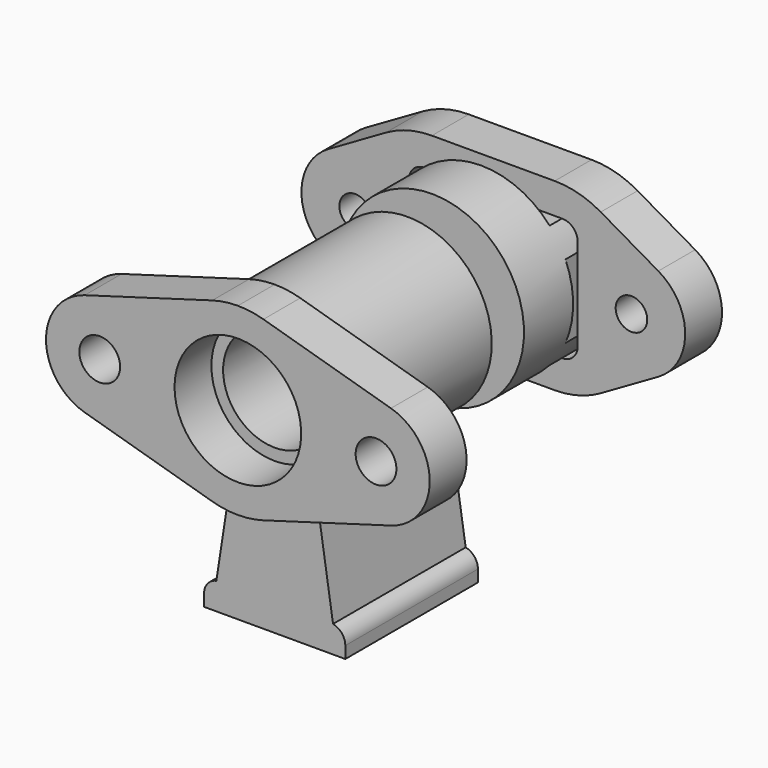
from build123d import *

# Parameters (mm, degrees)
F0_R      = 10.668
F1_DEPTH  = 34.29
F2_R      = 9.4615
F3_DEPTH  = 4.064
F5_D      = 6.5278
F5_DEPTH  = 19.05
F5_TIP    = 1.9611489744
F7_DEPTH  = 9.525
F8_D      = 26.19502
F9_D      = 8.4328
F11_R     = 19.05
F11_R_2   = 10.7823
F12_DEPTH = 25.4
F14_DEPTH = 12.7
F16_DEPTH = 9.525
F17_D     = 6.5278


# Not quite as in the source:
# - a pattern or mirror of a feature is missing from the dataset's text; its kind, count and spacing are read off the source's solid


with BuildPart() as f1:
    # F0 (on Front) → F1 (new body)
    with BuildSketch(Plane.XZ):
        with BuildLine():
            Line((12.065, -38.8341331818), (8.4555263158, -15.2788409565))
            ThreePointArc((8.4555263158, -15.2788409565), (0, 17.4625), (-8.4555263158, -15.2788409565))
            Line((-8.4555263158, -15.2788409565), (-12.065, -38.8341331818))
            ThreePointArc((-12.065, -38.8341331818), (-13.8893444248, -39.9369388409), (-14.605, -41.9449851551))
            Line((-14.605, -41.9449851551), (-14.605, -44.3992))
            Line((-14.605, -44.3992), (14.605, -44.3992))
            Line((14.605, -44.3992), (14.605, -41.9449851551))
            ThreePointArc((14.605, -41.9449851551), (13.8893444248, -39.9369388409), (12.065, -38.8341331818))
        make_face()
        Circle(F0_R, mode=Mode.SUBTRACT)
    extrude(amount=F1_DEPTH)

    # F2 (on face) → F3 (join)
    with BuildSketch(Plane(origin=(0, 0, -44.3992), x_dir=(1, 0, 0), z_dir=(0, 0, -1))):
        with Locations((0, 17.145)):
            Circle(F2_R)
    extrude(amount=F3_DEPTH)

    # F5
    with Locations(Plane(origin=(0, 0, -48.4632), x_dir=(1, 0, 0), z_dir=(0, 0, -1))):
        with Locations((0, 17.145)):
            Hole(F5_D / 2, depth=F5_DEPTH)
            with Locations((0, 0, -(F5_DEPTH + F5_TIP / 2))):  # 118° drill point
                Cone(0, F5_D / 2, F5_TIP, mode=Mode.SUBTRACT)


with BuildPart() as f7:
    # F6 (on face) → F7 (new body)
    with BuildSketch(Plane.XZ.offset(34.29)):
        with BuildLine():
            Line((5.2916666667, -18.300294093), (31.6618055556, -10.6751715542))
            ThreePointArc((31.6618055556, -10.6751715542), (39.6875, 0), (31.6618055556, 10.6751715542))
            Line((31.6618055556, 10.6751715542), (5.2916666667, 18.300294093))
            ThreePointArc((5.2916666667, 18.300294093), (2.6722553704, 18.861642326), (0, 19.05))
            ThreePointArc((0, 19.05), (-2.6722553704, 18.861642326), (-5.2916666667, 18.300294093))
            Line((-5.2916666667, 18.300294093), (-31.6618055556, 10.6751715542))
            ThreePointArc((-31.6618055556, 10.6751715542), (-39.6875, 0), (-31.6618055556, -10.6751715542))
            Line((-31.6618055556, -10.6751715542), (-5.2916666667, -18.300294093))
            ThreePointArc((-5.2916666667, -18.300294093), (-2.6722553704, -18.861642326), (0, -19.05))
            ThreePointArc((0, -19.05), (2.6722553704, -18.861642326), (5.2916666667, -18.300294093))
        make_face()
    extrude(amount=F7_DEPTH)

    # F8 (through all)
    with Locations(Plane(origin=(0, -34.29, 0), x_dir=(1, 0, 0), z_dir=(0, 1, 0))):
        with Locations((0, 0)):
            Hole(F8_D / 2)

    # F9 (through all)
    with Locations(Plane(origin=(0, -34.29, 0), x_dir=(1, 0, 0), z_dir=(0, 1, 0))):
        with Locations((28.575, 0), (-28.575, 0)):
            Hole(F9_D / 2)


with BuildPart() as f12:
    # F11 (on offset) → F12 (new body)
    with BuildSketch(Plane(origin=(0, 6.35, 0), x_dir=(-1, 0, 0), z_dir=(0, 1, 0))):
        Circle(F11_R)
        Circle(F11_R_2, mode=Mode.SUBTRACT)
    extrude(amount=F12_DEPTH)

    # F13 (on face) → F14 (cut)
    with BuildSketch(Plane(origin=(0, 31.75, 0), x_dir=(-1, 0, 0), z_dir=(0, 1, 0))):
        with BuildLine():
            Line((17.4625, 12.7), (14.1990316571, 12.7))
            ThreePointArc((14.1990316571, 12.7), (16.0337633139, 10.2869302512), (17.4625, 7.6133825433))
            Line((17.4625, 7.6133825433), (17.4625, 12.7))
        make_face()
        with BuildLine():
            Line((14.1990316571, -12.7), (-14.1990316571, -12.7))
            ThreePointArc((-14.1990316571, -12.7), (0, -19.05), (14.1990316571, -12.7))
        make_face()
        with BuildLine():
            Line((-17.4625, -7.6133825433), (-17.4625, 7.6133825433))
            ThreePointArc((-17.4625, 7.6133825433), (-19.05, 0), (-17.4625, -7.6133825433))
        make_face()
        with BuildLine():
            ThreePointArc((19.05, 0), (18.6489024476, 3.8885649667), (17.4625, 7.6133825433))
            Line((17.4625, 7.6133825433), (17.4625, -7.6133825433))
            ThreePointArc((17.4625, -7.6133825433), (18.6489024476, -3.8885649667), (19.05, 0))
        make_face()
    f14 = extrude(amount=-F14_DEPTH, mode=Mode.SUBTRACT)

    # F14_copies: F14 across plane
    add(f14.mirror(Plane.XY), mode=Mode.SUBTRACT)


with BuildPart() as f16:
    # F15 (on face) → F16 (new body)
    with BuildSketch(Plane(origin=(0, 31.75, 0), x_dir=(-1, 0, 0), z_dir=(0, 1, 0))):
        with BuildLine():
            Line((22.225, -16.4977839421), (34.13125, -9.6237072996))
            ThreePointArc((34.13125, -9.6237072996), (39.6875, 0), (34.13125, 9.6237072996))
            Line((34.13125, 9.6237072996), (22.225, 16.4977839421))
            ThreePointArc((22.225, 16.4977839421), (17.6305028092, 18.4008869908), (12.7, 19.05))
            Line((12.7, 19.05), (-12.7, 19.05))
            ThreePointArc((-12.7, 19.05), (-17.6305028092, 18.4008869908), (-22.225, 16.4977839421))
            Line((-22.225, 16.4977839421), (-34.13125, 9.6237072996))
            ThreePointArc((-34.13125, 9.6237072996), (-39.6875, 0), (-34.13125, -9.6237072996))
            Line((-34.13125, -9.6237072996), (-22.225, -16.4977839421))
            ThreePointArc((-22.225, -16.4977839421), (-17.6305028092, -18.4008869908), (-12.7, -19.05))
            Line((-12.7, -19.05), (12.7, -19.05))
            ThreePointArc((12.7, -19.05), (17.6305028092, -18.4008869908), (22.225, -16.4977839421))
        make_face()
        with BuildLine():
            ThreePointArc((-17.4625, 9.525), (-16.5325640303, 11.7700640303), (-14.2875, 12.7))
            Line((-14.2875, 12.7), (14.2875, 12.7))
            ThreePointArc((14.2875, 12.7), (16.5325640303, 11.7700640303), (17.4625, 9.525))
            Line((17.4625, 9.525), (17.4625, -9.525))
            ThreePointArc((17.4625, -9.525), (16.5325640303, -11.7700640303), (14.2875, -12.7))
            Line((14.2875, -12.7), (-14.2875, -12.7))
            ThreePointArc((-14.2875, -12.7), (-16.5325640303, -11.7700640303), (-17.4625, -9.525))
            Line((-17.4625, -9.525), (-17.4625, 9.525))
        make_face(mode=Mode.SUBTRACT)
    extrude(amount=-F16_DEPTH)

    # F17 (through all)
    with Locations(Plane(origin=(0, 31.75, 0), x_dir=(-1, 0, 0), z_dir=(0, 1, 0))):
        with Locations((-28.575, 0), (28.575, 0)):
            Hole(F17_D / 2)


solid = Compound([f1.part, f7.part, f12.part, f16.part])
